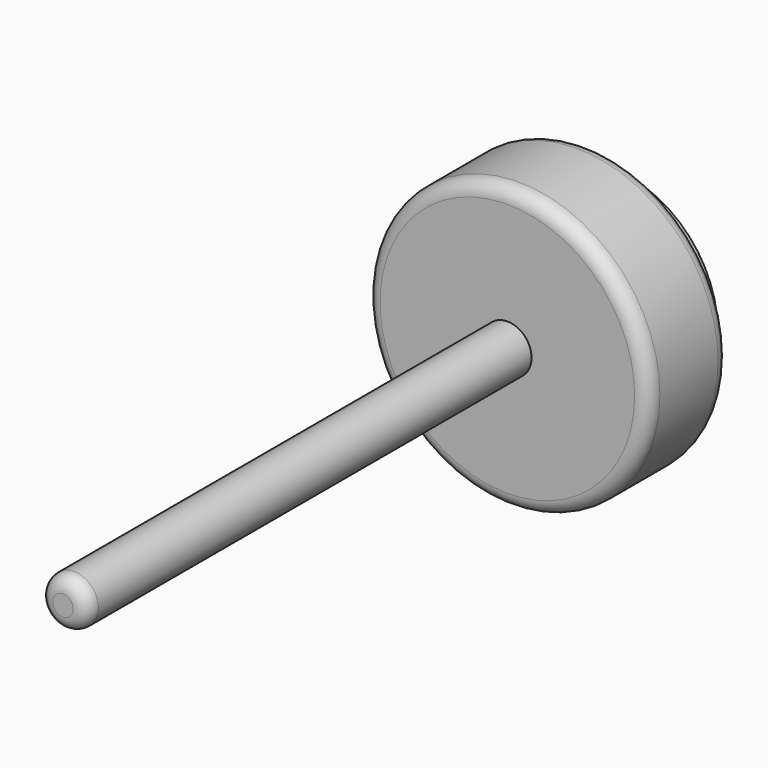
from build123d import *

# Parameters (mm, degrees)
F0_R         = 18.542
F1_DEPTH     = 13.208
F2_R         = 3.175
F3_DEPTH     = 86.106
F4_R         = 1.8396307345
F5_R         = 1.8396307345
F6_TEXT_SIZE = 10.4971501666
F7_DEPTH     = 3.048
F8_R         = 14.9205736619
F8_R_2       = 13.0364823299
F9_DEPTH     = 2.032
F10_R        = 14.1747090022
F10_R_2      = 13.749035402
F11_DEPTH    = 3.556
F12_S5_R     = 14.1747090022
F12_T6_DEPTH = 23
F14_DEPTH    = 2.54
F16_D        = 6.35
F16_DEPTH    = 18.543


# Not quite as in the source:
# - a fillet or chamfer that OpenCascade refuses, or shapes differently, is made with other operations: its cross-section is extruded or revolved along the edge and cut away or added
# - Text() gives the source's letters only with a copy of the font that has no kerning and outlines rounded to 1/6400 em; it was checked with that copy


with BuildPart() as f1:
    # F0 (on Front) → F1 (new body)
    with BuildSketch(Plane.XZ):
        Circle(F0_R)
    extrude(amount=F1_DEPTH)

    # F2 (on Front) → F3 (join)
    with BuildSketch(Plane.XZ):
        Circle(F2_R)
    extrude(amount=F3_DEPTH)

    # F4
    f4_edges = [f1.edges().sort_by_distance(p)[0] for p in [
        (-3.175, -86.106, 0),
    ]]
    fillet(f4_edges, radius=F4_R)

    # F5
    f5_edges = [f1.edges().sort_by_distance(p)[0] for p in [
        (-18.542, -13.208, 0),
        (-18.542, 0, 0),
    ]]
    fillet(f5_edges, radius=F5_R)

    # F6 (on Front) → F7 (cut)
    with BuildSketch(Plane.XZ):
        with Locations((-11.0448822379, -3.8538640365)):
            Text('.M.A', F6_TEXT_SIZE, font='Open Sans', text_align=(TextAlign.LEFT, TextAlign.BOTTOM))
    extrude(amount=F7_DEPTH, mode=Mode.SUBTRACT)

    # F8 (on Front) → F9 (join)
    with BuildSketch(Plane.XZ):
        Circle(F8_R)
        Circle(F8_R_2, mode=Mode.SUBTRACT)
    extrude(amount=-F9_DEPTH)

    # F10 (on Front) → F11 (join)
    with BuildSketch(Plane.XZ):
        Circle(F10_R)
        Circle(F10_R_2, mode=Mode.SUBTRACT)
    extrude(amount=-F11_DEPTH)

    # F12: chamfer of 1.016 on 1 edges, made by hand


with BuildPart() as f12_tool2:
    # F12_s3 → F12_t4 (revolve)
    with BuildSketch(Plane.XY):
        Polygon((14.9205736619, 1.016), (13.9045736619, 2.032), (14.9205736619, 2.032), align=None)
    revolve(axis=Axis((0, 2.032, 0), (0, -1, 0)))

    # F12_s5 → F12_t6 (cut, symmetric)
    with BuildSketch(Plane.XZ.offset(-1.5)):
        Circle(F12_S5_R)
    extrude(amount=F12_T6_DEPTH, both=True, mode=Mode.SUBTRACT)


with BuildPart() as f1_1:
    add(f1.part)

    # F12_t1: cut F12_tool2
    add(f12_tool2.part, mode=Mode.SUBTRACT)

    # F13 (on Front) → F14 (cut)
    with BuildSketch(Plane.XZ):
        with BuildLine():
            add(Edge.make_bspline(
                [(8.2746502012, 5.9290798381), (7.9746460411, 5.4817622812), (7.3549469124, 4.5577674267), (6.2082124493, 6.985085809), (3.9809270947, 2.804656653), (1.9952066907, 7.4019174607), (0.022451288, 2.9983474856), (-2.4887203534, 7.4603479972), (-5.0344602909, 3.0369553481), (-6.4575057704, 7.1563956587), (-8.0489305555, 4.3740950711), (-8.1231328636, 4.8740335025), (-8.1443395466, 5.0169136375)],
                knots=[0, 0, 0, 0, 0.0793432395, 0.1638941819, 0.2827612779, 0.3989064929, 0.5120701546, 0.6349951678, 0.7564961992, 0.8637195611, 0.961051669, 1, 1, 1, 1], degree=3))
            add(Edge.make_bspline(
                [(-8.1443395466, 5.0169136375), (-7.7105370502, 5.9969196759), (-6.8255534975, 7.9961917702), (-4.6531673364, 3.7573085347), (-2.5873577992, 8.881869254), (-0.3078596292, 3.7858636073), (2.1409600621, 9.5534027576), (4.0444961427, 2.9144835376), (6.0048279519, 8.4621773144), (7.3658534369, 5.5278428062), (8.0159089361, 5.8148446413), (8.2746502012, 5.9290798381)],
                knots=[0, 0, 0, 0, 0.1090921286, 0.2225545965, 0.3442937694, 0.4633701681, 0.5881219717, 0.7172060621, 0.8385762918, 0.9357486022, 1, 1, 1, 1], degree=3))
        make_face()
        with BuildLine():
            add(Edge.make_bspline(
                [(8.2746502012, -5.9290798381), (7.9746460411, -5.4817622812), (7.3549469124, -4.5577674267), (6.2082124493, -6.985085809), (3.9809270947, -2.804656653), (1.9952066907, -7.4019174607), (0.022451288, -2.9983474856), (-2.4887203534, -7.4603479972), (-5.0344602909, -3.0369553481), (-6.4575057704, -7.1563956587), (-8.0489305555, -4.3740950711), (-8.1231328636, -4.8740335025), (-8.1443395466, -5.0169136375)],
                knots=[0, 0, 0, 0, 0.0793432395, 0.1638941819, 0.2827612779, 0.3989064929, 0.5120701546, 0.6349951678, 0.7564961992, 0.8637195611, 0.961051669, 1, 1, 1, 1], degree=3))
            add(Edge.make_bspline(
                [(-8.1443395466, -5.0169136375), (-7.7105370502, -5.9969196759), (-6.8255534975, -7.9961917702), (-4.6531673364, -3.7573085347), (-2.5873577992, -8.881869254), (-0.3078596292, -3.7858636073), (2.1409600621, -9.5534027576), (4.0444961427, -2.9144835376), (6.0048279519, -8.4621773144), (7.3658534369, -5.5278428062), (8.0159089361, -5.8148446413), (8.2746502012, -5.9290798381)],
                knots=[0, 0, 0, 0, 0.1090921286, 0.2225545965, 0.3442937694, 0.4633701681, 0.5881219717, 0.7172060621, 0.8385762918, 0.9357486022, 1, 1, 1, 1], degree=3))
        make_face()
    extrude(amount=F14_DEPTH, mode=Mode.SUBTRACT)

    # F16 (through all, one way)
    with BuildSketch(Plane.XY):
        with Locations((0, -5.8550667018)):
            Circle(F16_D / 2)
    extrude(amount=-F16_DEPTH, mode=Mode.SUBTRACT)


solid = f1_1.part
